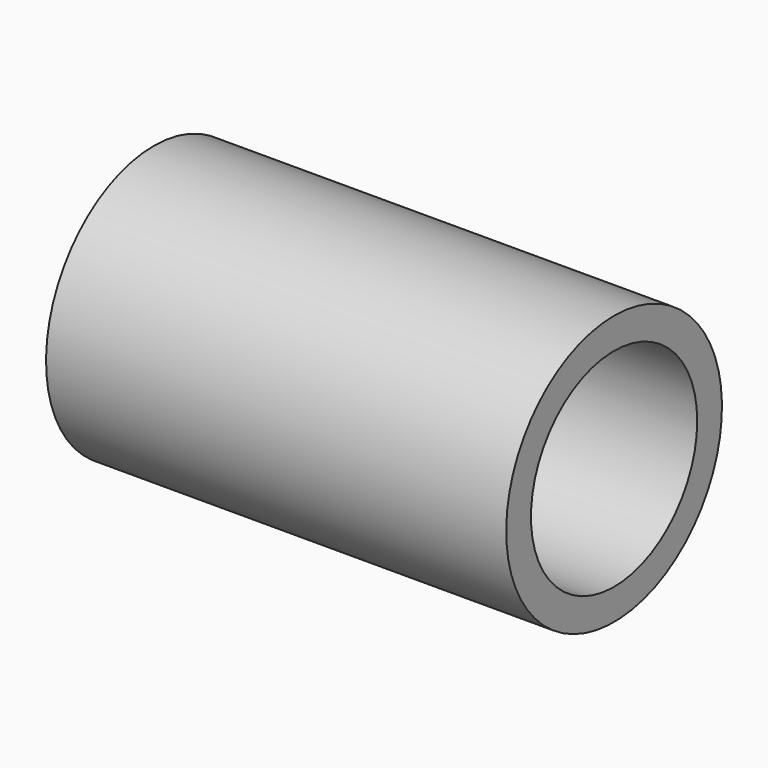
from build123d import *

# Parameters (mm, degrees)
F0_W     = 47.244
F0_H     = 13.843
F2_R     = 10.668
F3_DEPTH = 47.244


# Not quite as in the source:
# - a feature names something its author has since deleted; it is built from what else it names


with BuildPart() as f1:
    # F0 (on Front) → F1 (revolve)
    with BuildSketch(Plane.XZ):
        with Locations((23.622, 6.9215)):
            Rectangle(F0_W, F0_H)
    revolve(axis=Axis((23.622, 0, 0), (1, 0, 0)))

    # F2 (on face) → F3 (cut, through all)
    with BuildSketch(Plane.YZ.offset(47.244)):
        Circle(F2_R)
    extrude(amount=-F3_DEPTH, mode=Mode.SUBTRACT)


solid = f1.part
